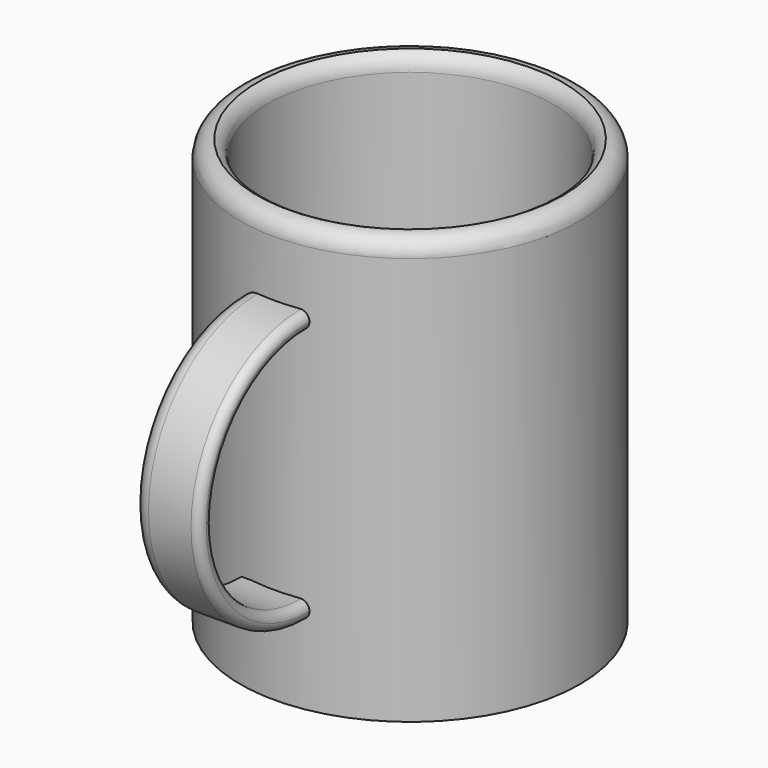
from build123d import *

# Parameters (mm, degrees)
F0_R          = 50
F1_DEPTH      = 125
F2_T          = -8
F3_R          = 5
F6_DEPTH      = 10
F6_DEPTH_BACK = 10
F7_R          = 2.5
F8_R          = 2.49999
F9_R          = 4.99999


# Not quite as in the source:
# - a fillet or chamfer that OpenCascade refuses, or shapes differently, is made with other operations: its cross-section is extruded or revolved along the edge and cut away or added
# - a fillet or chamfer is up to 0.001 mm smaller than in the source, because OpenCascade refuses the exact size


with BuildPart() as f1:
    # F0 (on Top) → F1 (new body)
    with BuildSketch(Plane.XY):
        Circle(F0_R)
    extrude(amount=F1_DEPTH)

    # F2
    f2_openings = [f1.faces().sort_by_distance(p)[0] for p in [
        (0, 0, 125),
    ]]
    offset(amount=F2_T, openings=f2_openings)

    # F3
    f3_edges = [f1.edges().sort_by_distance(p)[0] for p in [
        (-50, 0, 125),
    ]]
    fillet(f3_edges, radius=F3_R)

    # F4: fillet of radius 5 on 1 edges, made by hand

    # F4_s1 → F4_t2 (revolve, cut)
    with BuildSketch(Plane.XZ):
        with BuildLine():
            ThreePointArc((45, 125), (42.8166998673, 123.1560370926), (42, 120.417424305))
            Line((42, 120.417424305), (42, 125))
            Line((42, 125), (45, 125))
        make_face()
    revolve(axis=Axis((0, 0, 125), (0, 0, 1)), mode=Mode.SUBTRACT)

    # F5 (on Right) → F6 (join, two sides)
    with BuildSketch(Plane.YZ) as f6_sk:
        with BuildLine():
            ThreePointArc((-49.5038208311, 28.4888988916), (-84.9579082425, 63.4859531194), (-49.5038208311, 98.4830073472))
            Line((-49.5038208311, 98.4830073472), (-49.5038208311, 103.4833755941))
            ThreePointArc((-49.5038208311, 103.4833755941), (-89.9579082425, 63.4859531194), (-49.5038208311, 23.4885306446))
            Line((-49.5038208311, 23.4885306446), (-49.5038208311, 28.4888988916))
        make_face()
    extrude(amount=F6_DEPTH)
    extrude(f6_sk.sketch, amount=-F6_DEPTH_BACK)

    # F7
    f7_edges = [f1.edges().sort_by_distance(p)[0] for p in [
        (10, -89.957908, 63.485953),
    ]]
    fillet(f7_edges, radius=F7_R)

    # F8 (radius 2.5 in the source; OpenCascade refuses exactly that, so slightly less here)
    f8_edges = [f1.edges().sort_by_distance(p)[0] for p in [
        (10, -84.957908, 63.485953),
    ]]
    fillet(f8_edges, radius=F8_R)

    # F9 (radius 5 in the source; OpenCascade refuses exactly that, so slightly less here)
    f9_edges = [f1.edges().sort_by_distance(p)[0] for p in [
        (-10, -89.957908, 63.485953),
    ]]
    fillet(f9_edges, radius=F9_R)


solid = f1.part
